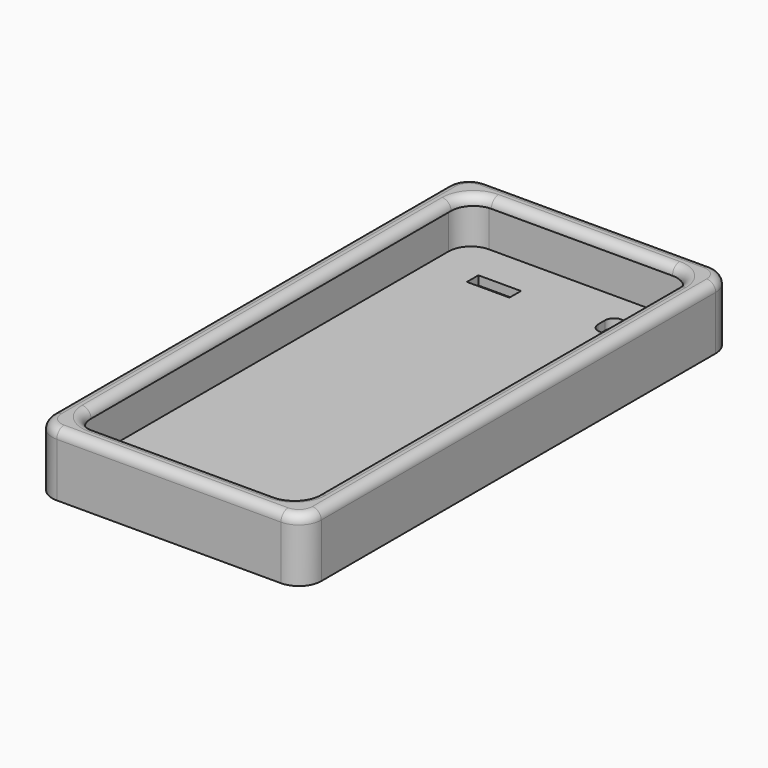
from build123d import *

# Parameters (mm, degrees)
F0_W      = 152.4
F0_H      = 304.8
F1_DEPTH  = 5.08
F2_W      = 152.4
F2_H      = 304.8
F2_W_2    = 142.2399785995
F2_H_2    = 294.6399785995
F3_DEPTH  = 25.4
F4_W      = 152.4
F4_H      = 304.8
F4_W_2    = 142.2399785995
F4_H_2    = 294.6399785995
F4_W_3    = 128.0160005927
F4_H_3    = 280.4160005927
F5_DEPTH  = 5.08
F6_R      = 12.7
F7_W      = 32.2413705289
F7_H      = 15.166670084
F8_DEPTH  = 25.4
F9_R      = 5.07999
F10_W     = 24.1091474891
F10_H     = 8.1412196159
F11_DEPTH = 25.4


# Not quite as in the source:
# - a fillet or chamfer is up to 0.001 mm smaller than in the source, because OpenCascade refuses the exact size


with BuildPart() as f1:
    # F0 (on Top) → F1 (new body)
    with BuildSketch(Plane.XY):
        with Locations((-76.2, 152.4)):
            Rectangle(F0_W, F0_H)
    extrude(amount=F1_DEPTH)

    # F2 (on face) → F3 (join)
    with BuildSketch(Plane.XY.offset(5.08)):
        with Locations((-76.2, 152.4)):
            Rectangle(F2_W, F2_H)
        with Locations((-76.2, 152.4)):
            Rectangle(F2_W_2, F2_H_2, mode=Mode.SUBTRACT)
    extrude(amount=F3_DEPTH)

    # F4 (on face) → F5 (join)
    with BuildSketch(Plane.XY.offset(30.48)):
        with Locations((-76.2, 152.4)):
            Rectangle(F4_W, F4_H)
        with Locations((-76.2, 152.4)):
            Rectangle(F4_W_2, F4_H_2, mode=Mode.SUBTRACT)
        with Locations((-76.2, 152.4)):
            Rectangle(F4_W_2, F4_H_2)
        with Locations((-76.2, 152.4)):
            Rectangle(F4_W_3, F4_H_3, mode=Mode.SUBTRACT)
    extrude(amount=F5_DEPTH)

    # F6
    f6_edges = [f1.edges().sort_by_distance(p)[0] for p in [
        (-152.4, 0, 17.78),
        (0, 0, 17.78),
        (0, 304.8, 17.78),
        (-152.4, 304.8, 17.78),
        (-147.319989, 5.080011, 17.78),
        (-5.080011, 5.080011, 17.78),
        (-5.080011, 299.719989, 17.78),
        (-147.319989, 299.719989, 17.78),
        (-140.208, 12.192, 33.02),
        (-12.192, 292.608, 33.02),
        (-140.208, 292.608, 33.02),
        (-12.192, 12.192, 33.02),
    ]]
    fillet(f6_edges, radius=F6_R)

    # F7 (on face) → F8 (cut)
    with BuildSketch(Plane(origin=(0, 0, 0), x_dir=(1, 0, 0), z_dir=(0, 0, -1))):
        with Locations((-35.8565431088, -276.2855738401)):
            Rectangle(F7_W, F7_H)
    extrude(amount=-F8_DEPTH, mode=Mode.SUBTRACT)

    # F9 (radius 5.08 in the source; OpenCascade refuses exactly that, so slightly less here)
    f9_edges = [f1.edges().sort_by_distance(p)[0] for p in [
        (-51.977228, 283.868909, 2.54),
        (-19.735858, 283.868909, 2.54),
        (-19.735858, 268.702239, 2.54),
        (-51.977228, 268.702239, 2.54),
        (-76.2, 304.8, 35.56),
        (-3.719744, 301.080256, 35.56),
        (-148.680256, 301.080256, 35.56),
        (0, 152.4, 35.56),
        (-152.4, 152.4, 35.56),
        (-3.719744, 3.719744, 35.56),
        (-148.680256, 3.719744, 35.56),
        (-76.2, 0, 35.56),
        (-140.208, 152.4, 35.56),
        (-136.488256, 15.911744, 35.56),
        (-136.488256, 288.888256, 35.56),
        (-76.2, 12.192, 35.56),
        (-76.2, 292.608, 35.56),
        (-15.911744, 15.911744, 35.56),
        (-15.911744, 288.888256, 35.56),
        (-12.192, 152.4, 35.56),
    ]]
    fillet(f9_edges, radius=F9_R)

    # F10 (on face) → F11 (cut)
    with BuildSketch(Plane(origin=(0, 0, 0), x_dir=(1, 0, 0), z_dir=(0, 0, -1))):
        with Locations((-110.6483452022, -273.3389437199)):
            Rectangle(F10_W, F10_H)
    extrude(amount=-F11_DEPTH, mode=Mode.SUBTRACT)


solid = f1.part
